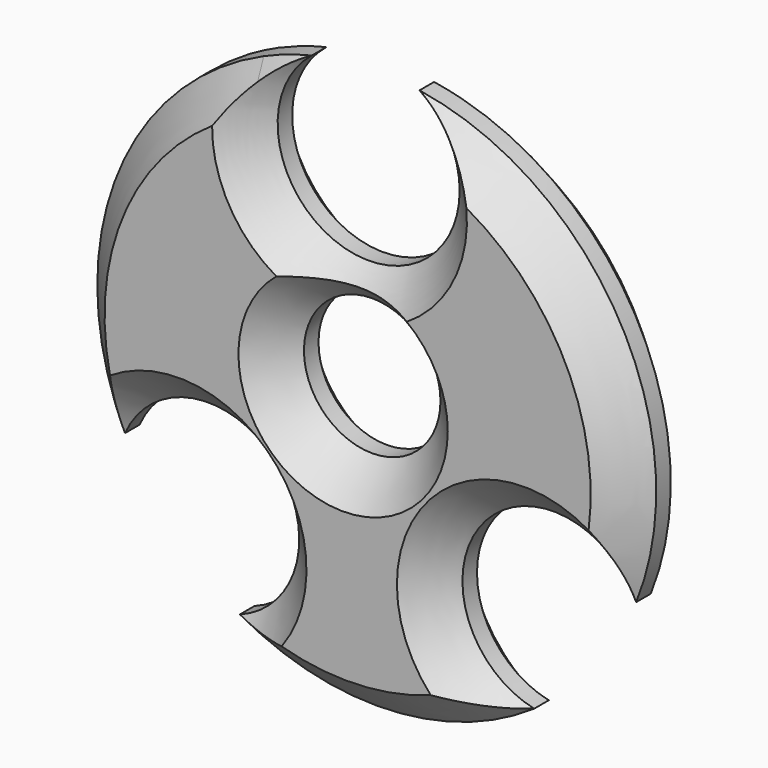
from build123d import *
from build123d import SkipClean  # not in build123d's __all__

# Parameters (mm, degrees)
F0_R         = 38.997292
F2_DEPTH     = 12.7
F3_D         = 25.4
F5_D         = 19.05
F6_T2_ANGLE  = 351.374344
F6_T4_ANGLE  = 102.020033
F6_T6_ANGLE  = 154.888124
F6_T8_ANGLE  = 343.872337
F6_T10_ANGLE = 359.64
F6_T12_ANGLE = 154.152245
F7_T2_ANGLE  = 154.888124
F7_T4_ANGLE  = 351.374344
F7_T6_ANGLE  = 359.64
F7_T8_ANGLE  = 102.020033
F7_T10_ANGLE = 154.152245
F7_T12_ANGLE = 343.872337


# Not quite as in the source:
# - a fillet or chamfer that OpenCascade refuses, or shapes differently, is made with other operations: its cross-section is extruded or revolved along the edge and cut away or added


with BuildPart() as f2:
    # F0 (on Front) → F2 (new body)
    with BuildSketch(Plane.XZ):
        with Locations((-14.654592, 18.190622)):
            Circle(F0_R)
    extrude(amount=F2_DEPTH)

    # F3 (through all)
    with Locations(Plane(origin=(0, 0, 0), x_dir=(1, 0, 0), z_dir=(0, 1, 0))):
        with Locations((-15.788088, -46.200868), (-38.174681, 3.901272), (9.999, 1.613084)):
            Hole(F3_D / 2)

    # F5 (through all)
    with Locations(Plane.XZ.offset(12.7)):
        with Locations((-15.289431, 19.513205)):
            Hole(F5_D / 2)

    # F6: chamfer of 5.08 on 7 edges, made by hand

    # F6_s1 → F6_t2 (revolve, cut)
    with BuildSketch(Plane(origin=(3.861156, 0, 4.127998), x_dir=(0, 1, 0), z_dir=(0.683108, 0, 0.730317))):
        Polygon((-7.62, -21.104353), (-12.7, -26.184353), (-12.7, -21.104353), align=None)
    revolve(axis=Axis((9.999, -12.7, -1.613084), (0, 1, 0)), revolution_arc=F6_T2_ANGLE, mode=Mode.SUBTRACT)

    # F6_s3 → F6_t4 (revolve, cut)
    with BuildSketch(Plane(origin=(-15.453869, 0, 17.484158), x_dir=(0, 1, 0), z_dir=(-0.662264, 0, 0.749271))):
        Polygon((-12.7, 32.850552), (-7.62, 37.930552), (-12.7, 37.930552), align=None)
    revolve(axis=Axis((-14.654592, -12.7, 18.190622), (0, -1, 0)), revolution_arc=F6_T4_ANGLE, mode=Mode.SUBTRACT)

    # F6_s5 → F6_t6 (revolve, cut)
    with BuildSketch(Plane(origin=(-5.535221, 0, -2.446024), x_dir=(0, 1, 0), z_dir=(-0.914673, 0, -0.404195))):
        Polygon((-7.62, -61.559076), (-12.7, -56.479076), (-12.7, -61.559076), align=None)
    revolve(axis=Axis((-14.654592, -12.7, 18.190622), (0, 1, 0)), revolution_arc=F6_T6_ANGLE, mode=Mode.SUBTRACT)

    # F6_s7 → F6_t8 (revolve, cut)
    with BuildSketch(Plane(origin=(-10.812222, 0, 15.35988), x_dir=(0, 1, 0), z_dir=(0.575615, 0, -0.817721))):
        Polygon((-12.7, -51.241861), (-7.62, -46.161861), (-12.7, -46.161861), align=None)
    revolve(axis=Axis((-38.174681, -12.7, -3.901272), (0, 1, 0)), revolution_arc=F6_T8_ANGLE, mode=Mode.SUBTRACT)

    # F6_s9 → F6_t10 (revolve, cut)
    with BuildSketch(Plane(origin=(-13.746918, 0, -0.599563), x_dir=(0, 1, 0), z_dir=(0.99905, 0, 0.043573))):
        Polygon((-12.7, 64.624921), (-7.62, 59.544921), (-12.7, 59.544921), align=None)
    revolve(axis=Axis((-15.788088, -12.7, 46.200868), (0, -1, 0)), revolution_arc=F6_T10_ANGLE, mode=Mode.SUBTRACT)

    # F6_s11 → F6_t12 (revolve, cut)
    with BuildSketch(Plane(origin=(-18.719704, 0, 6.521018), x_dir=(0, 1, 0), z_dir=(0.944343, 0, -0.328962))):
        Polygon((-12.7, 46.274671), (-7.62, 51.354671), (-12.7, 51.354671), align=None)
    with SkipClean():  # cleaning this boolean's faces spoils the solid; the shape is the same uncleaned
        revolve(axis=Axis((-14.654592, -12.7, 18.190622), (0, -1, 0)), revolution_arc=F6_T12_ANGLE, mode=Mode.SUBTRACT)

    # F6_s13 → F6_t14 (revolve, cut)
    with BuildSketch(Plane.XY.offset(19.513205)):
        Polygon((-0.684431, -12.7), (-5.764431, -7.62), (-5.764431, -12.7), align=None)
    revolve(axis=Axis((-15.289431, -12.7, 19.513205), (0, -1, 0)), mode=Mode.SUBTRACT)

    # F7: chamfer of 5.08 on 7 edges, made by hand

    # F7_s1 → F7_t2 (revolve, cut)
    with BuildSketch(Plane(origin=(2.689337, 0, 3.088564), x_dir=(0, 1, 0), z_dir=(-0.656683, 0, -0.754167))):
        Polygon((-5.08, 15.999814), (0, 10.919814), (0, 15.999814), align=None)
    revolve(axis=Axis((-14.654592, 0, 18.190622), (0, -1, 0)), revolution_arc=F7_T2_ANGLE, mode=Mode.SUBTRACT)

    # F7_s3 → F7_t4 (revolve, cut)
    with BuildSketch(Plane(origin=(3.861156, 0, 4.127998), x_dir=(0, 1, 0), z_dir=(0.683108, 0, 0.730317))):
        Polygon((-5.08, -21.104353), (0, -26.184353), (0, -21.104353), align=None)
    revolve(axis=Axis((9.999, 0, -1.613084), (0, 1, 0)), revolution_arc=F7_T4_ANGLE, mode=Mode.SUBTRACT)

    # F7_s5 → F7_t6 (revolve, cut)
    with BuildSketch(Plane(origin=(-13.746918, 0, -0.599563), x_dir=(0, 1, 0), z_dir=(0.99905, 0, 0.043573))):
        Polygon((-5.08, 59.544921), (0, 64.624921), (0, 59.544921), align=None)
    revolve(axis=Axis((-15.788088, 0, 46.200868), (0, -1, 0)), revolution_arc=F7_T6_ANGLE, mode=Mode.SUBTRACT)

    # F7_s7 → F7_t8 (revolve, cut)
    with BuildSketch(Plane(origin=(-15.453869, 0, 17.484158), x_dir=(0, 1, 0), z_dir=(-0.662264, 0, 0.749271))):
        Polygon((-5.08, 37.930552), (0, 32.850552), (0, 37.930552), align=None)
    revolve(axis=Axis((-14.654592, 0, 18.190622), (0, -1, 0)), revolution_arc=F7_T8_ANGLE, mode=Mode.SUBTRACT)

    # F7_s9 → F7_t10 (revolve, cut)
    with BuildSketch(Plane(origin=(-18.719704, 0, 6.521018), x_dir=(0, 1, 0), z_dir=(0.944343, 0, -0.328962))):
        Polygon((-5.08, 51.354671), (0, 46.274671), (0, 51.354671), align=None)
    revolve(axis=Axis((-14.654592, 0, 18.190622), (0, -1, 0)), revolution_arc=F7_T10_ANGLE, mode=Mode.SUBTRACT)

    # F7_s11 → F7_t12 (revolve, cut)
    with BuildSketch(Plane(origin=(-21.327756, 0, 17.104865), x_dir=(0, 1, 0), z_dir=(-0.780107, 0, 0.625646))):
        Polygon((-5.08, 39.627247), (0, 44.707247), (0, 39.627247), align=None)
    revolve(axis=Axis((-38.174681, 0, -3.901272), (0, -1, 0)), revolution_arc=F7_T12_ANGLE, mode=Mode.SUBTRACT)

    # F7_s13 → F7_t14 (revolve, cut)
    with BuildSketch(Plane.XY.offset(19.513205)):
        Polygon((-5.764431, -5.08), (-0.684431, 0), (-5.764431, 0), align=None)
    revolve(axis=Axis((-15.289431, 0, 19.513205), (0, -1, 0)), mode=Mode.SUBTRACT)


solid = f2.part
